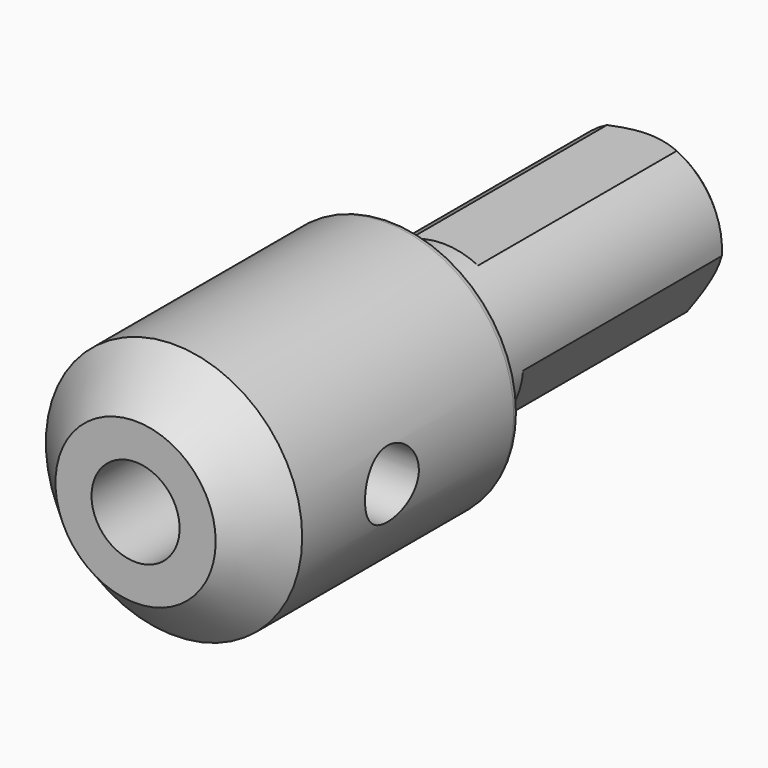
from build123d import *

# Parameters (mm, degrees)
F0_R            = 8
F1_DEPTH        = 20
F2_R            = 5
F3_DEPTH        = 20
F5_DEPTH        = 16
F5_COPIES_COUNT = 3
F6_SIZE         = 0.49999
F7_R            = 0.5
F9_D            = 5.5
F9_DEPTH        = 14
F9_TIP          = 1.6523667023
F10_R           = 2.1
F11_DEPTH       = 8.25
F12_SIZE        = 3


# Not quite as in the source:
# - a fillet or chamfer is up to 0.001 mm smaller than in the source, because OpenCascade refuses the exact size
# - a pattern or mirror of a feature is missing from the dataset's text; its kind, count and spacing are read off the source's solid


with BuildPart() as f1:
    # F0 (on Front) → F1 (new body)
    with BuildSketch(Plane.XZ):
        Circle(F0_R)
    extrude(amount=-F1_DEPTH)

    # F2 (on face) → F3 (join)
    with BuildSketch(Plane(origin=(0, 20, 0), x_dir=(-1, 0, 0), z_dir=(0, 1, 0))):
        Circle(F2_R)
    extrude(amount=F3_DEPTH)

    # F4 (on face) → F5 (cut)
    with BuildSketch(Plane(origin=(0, 40, 0), x_dir=(-1, 0, 0), z_dir=(0, 1, 0))):
        with BuildLine():
            ThreePointArc((2.1794494718, 4.5), (0, 5), (-2.1794494718, 4.5))
            Line((-2.1794494718, 4.5), (2.1794494718, 4.5))
        make_face()
    f5 = extrude(amount=-F5_DEPTH, mode=Mode.SUBTRACT)

    # F5_copies: F5 ×3 about axis
    f5_copies_axis = Axis((0, 0, 0), (0, 1, 0))
    for i in range(1, F5_COPIES_COUNT):
        add(f5.rotate(f5_copies_axis, i * 360 / F5_COPIES_COUNT), mode=Mode.SUBTRACT)

    # F6 (size 0.5 in the source; OpenCascade refuses exactly that, so slightly less here)
    f6_edges = [f1.edges().sort_by_distance(p)[0] for p in [
        (4.330127, 40, 2.5),
        (-4.996709, 40, -0.18139),
        (0, 40, -5),
        (-4.236582, 40, 2.655443),
    ]]
    chamfer(f6_edges, length=F6_SIZE)

    # F7
    f7_edges = [f1.edges().sort_by_distance(p)[0] for p in [
        (-8, 20, 0),
        (5, 20, 0),
    ]]
    fillet(f7_edges, radius=F7_R)

    # F9
    with Locations(Plane.XZ):
        with Locations((0, 0)):
            Hole(F9_D / 2, depth=F9_DEPTH)
            with Locations((0, 0, -(F9_DEPTH + F9_TIP / 2))):  # 118° drill point
                Cone(0, F9_D / 2, F9_TIP, mode=Mode.SUBTRACT)

    # F10 (on Right) → F11 (cut, symmetric)
    with BuildSketch(Plane.YZ):
        with Locations((10, 0)):
            Circle(F10_R)
    extrude(amount=F11_DEPTH, both=True, mode=Mode.SUBTRACT)

    # F12
    f12_edges = [f1.edges().sort_by_distance(p)[0] for p in [
        (-8, 0, 0),
    ]]
    chamfer(f12_edges, length=F12_SIZE)


solid = f1.part
